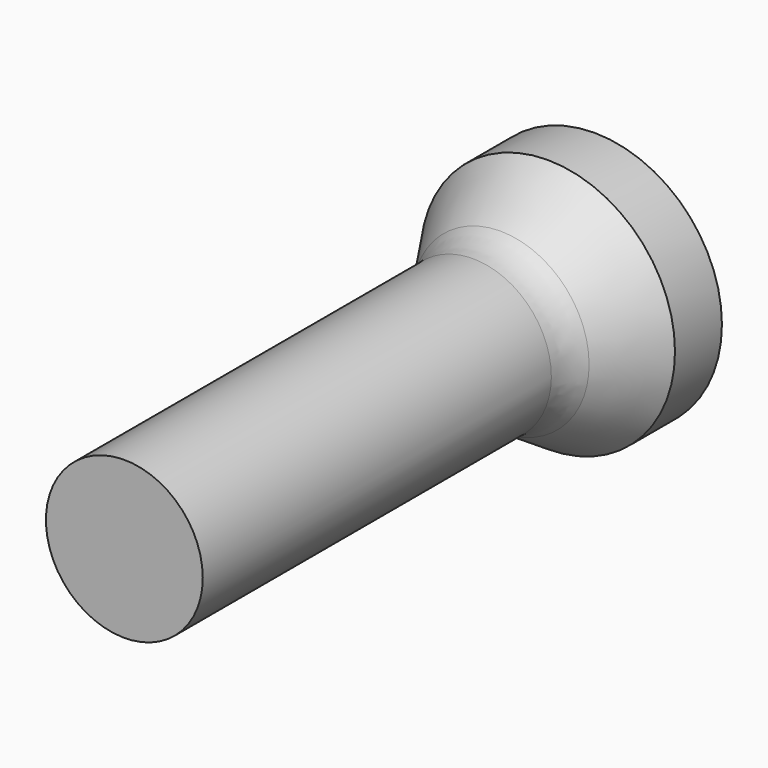
from build123d import *

# Parameters (mm, degrees)
F0_R     = 6.35
F1_DEPTH = 42.8498
F0_R_2   = 10.3124
F2_DEPTH = 4.7498
F5_R     = 6.35
F6_R     = 10.3124
F8_R     = 5.08


with BuildPart() as f1:
    # F0 (on Front) → F1 (new body)
    with BuildSketch(Plane.XZ):
        Circle(F0_R)
    extrude(amount=F1_DEPTH)

    # F5 (on plane+point) → F7 section 0
    with BuildSketch(Plane.XZ.offset(6.0488656163)):
        Circle(F5_R)
    # F6 (on Front) → F7 section 1
    with BuildSketch(Plane.XZ):
        Circle(F6_R)
    loft()

    # F8
    f8_edges = [f1.edges().sort_by_distance(p)[0] for p in [
        (-6.35, -6.048866, 0),
    ]]
    fillet(f8_edges, radius=F8_R)


with BuildPart() as f2:
    # F0 (on Front) → F2 (new body)
    with BuildSketch(Plane.XZ):
        Circle(F0_R_2)
        Circle(F0_R, mode=Mode.SUBTRACT)
        Circle(F0_R)
    extrude(amount=-F2_DEPTH)


solid = Compound([f1.part, f2.part])
